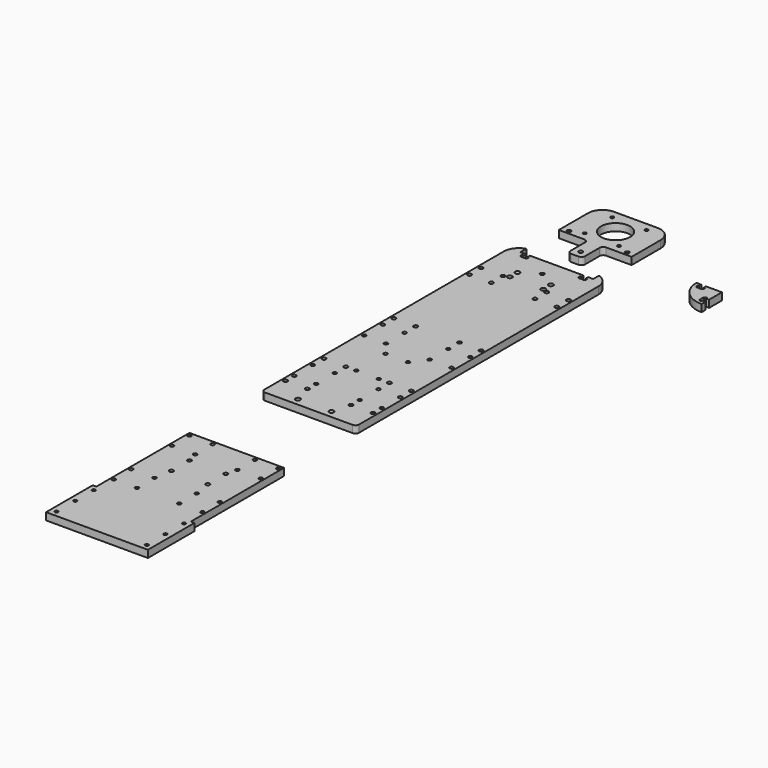
from build123d import *

# Parameters (mm, degrees)
F0_R     = 2.75
F0_R_2   = 2.5
F0_R_3   = 3.3
F1_DEPTH = 10
F0_W     = 130
F0_H     = 140
F0_H_2   = 20
F0_H_3   = 80
F0_R_4   = 2.25
F0_W_2   = 5
F2_DEPTH = 10
F0_R_5   = 20
F3_DEPTH = 10
F4_DEPTH = 10


# Not quite as in the source:
# - a feature names something its author has since deleted; it is built from what else it names


with BuildPart() as f1:
    # F0 (on Top) → F1 (new body)
    with BuildSketch(Plane.XY):
        with BuildLine():
            Line((65, 200), (-65, 200))
            Line((-65, 200), (-65, -121))
            ThreePointArc((-65, -121), (-63.5355339059, -124.5355339059), (-60, -126))
            Line((-60, -126), (60, -126))
            ThreePointArc((60, -126), (63.5355339059, -124.5355339059), (65, -121))
            Line((65, -121), (65, 200))
        make_face()
        with Locations((-60, -91)):
            Circle(F0_R, mode=Mode.SUBTRACT)
        with Locations((-60, -76)):
            Circle(F0_R_2, mode=Mode.SUBTRACT)
        with Locations((-60, -44)):
            Circle(F0_R_2, mode=Mode.SUBTRACT)
        with Locations((-30, -91)):
            Circle(F0_R, mode=Mode.SUBTRACT)
        with Locations((-23, -116)):
            Circle(F0_R_3, mode=Mode.SUBTRACT)
        with Locations((-30, -76)):
            Circle(F0_R_2, mode=Mode.SUBTRACT)
        with Locations((-30, -44)):
            Circle(F0_R_2, mode=Mode.SUBTRACT)
        with Locations((23, -116)):
            Circle(F0_R_3, mode=Mode.SUBTRACT)
        with Locations((30, -91)):
            Circle(F0_R, mode=Mode.SUBTRACT)
        with Locations((30, -76)):
            Circle(F0_R_2, mode=Mode.SUBTRACT)
        with Locations((30, -44)):
            Circle(F0_R_2, mode=Mode.SUBTRACT)
        with Locations((60, -91)):
            Circle(F0_R, mode=Mode.SUBTRACT)
        with Locations((60, -76)):
            Circle(F0_R_2, mode=Mode.SUBTRACT)
        with Locations((60, -44)):
            Circle(F0_R_2, mode=Mode.SUBTRACT)
        with Locations((-60, -25)):
            Circle(F0_R, mode=Mode.SUBTRACT)
        with Locations((-60, 44)):
            Circle(F0_R_2, mode=Mode.SUBTRACT)
        with Locations((-60, 76)):
            Circle(F0_R_2, mode=Mode.SUBTRACT)
        with Locations((-30, -25)):
            Circle(F0_R, mode=Mode.SUBTRACT)
        with Locations((-15.5, -25)):
            Circle(F0_R_2, mode=Mode.SUBTRACT)
        with Locations((-15.5, 25)):
            Circle(F0_R_2, mode=Mode.SUBTRACT)
        with Locations((-30, 44)):
            Circle(F0_R_2, mode=Mode.SUBTRACT)
        with Locations((-30, 76)):
            Circle(F0_R_2, mode=Mode.SUBTRACT)
        with Locations((-60, 95)):
            Circle(F0_R, mode=Mode.SUBTRACT)
        with Locations((-30, 95)):
            Circle(F0_R, mode=Mode.SUBTRACT)
        with Locations((15.5, -25)):
            Circle(F0_R_2, mode=Mode.SUBTRACT)
        with Locations((15.5, 25)):
            Circle(F0_R_2, mode=Mode.SUBTRACT)
        with Locations((30, -25)):
            Circle(F0_R, mode=Mode.SUBTRACT)
        with Locations((30, 44)):
            Circle(F0_R_2, mode=Mode.SUBTRACT)
        with Locations((30, 76)):
            Circle(F0_R_2, mode=Mode.SUBTRACT)
        with Locations((30, 95)):
            Circle(F0_R, mode=Mode.SUBTRACT)
        with Locations((60, -25)):
            Circle(F0_R, mode=Mode.SUBTRACT)
        with Locations((60, 44)):
            Circle(F0_R_2, mode=Mode.SUBTRACT)
        with Locations((60, 76)):
            Circle(F0_R_2, mode=Mode.SUBTRACT)
        with Locations((60, 95)):
            Circle(F0_R, mode=Mode.SUBTRACT)
        with BuildLine():
            Line((-65, 290), (-65, 200))
            Line((-65, 200), (65, 200))
            Line((65, 200), (65, 290))
            ThreePointArc((65, 290), (62.0710678119, 297.0710678119), (55, 300))
            Line((55, 300), (50, 300))
            Line((50, 300), (43, 300))
            Line((43, 300), (43, 296))
            Line((43, 296), (45, 296))
            Line((45, 296), (45, 293.6))
            Line((45, 293.6), (43.4, 292))
            Line((43.4, 292), (40, 292))
            Line((40, 292), (36.6, 292))
            Line((36.6, 292), (35, 293.6))
            Line((35, 293.6), (35, 296))
            Line((35, 296), (37, 296))
            Line((37, 296), (37, 300))
            Line((37, 300), (-37, 300))
            Line((-37, 300), (-37, 296))
            Line((-37, 296), (-35, 296))
            Line((-35, 296), (-35, 293.6))
            Line((-35, 293.6), (-36.6, 292))
            Line((-36.6, 292), (-37.5, 292))
            Line((-37.5, 292), (-40, 292))
            Line((-40, 292), (-42.5, 292))
            Line((-42.5, 292), (-43.4, 292))
            Line((-43.4, 292), (-45, 293.6))
            Line((-45, 293.6), (-45, 296))
            Line((-45, 296), (-43, 296))
            Line((-43, 296), (-43, 300))
            Line((-43, 300), (-50, 300))
            Line((-50, 300), (-55, 300))
            ThreePointArc((-55, 300), (-62.0710678119, 297.0710678119), (-65, 290))
        make_face()
        with Locations((-60, 225)):
            Circle(F0_R, mode=Mode.SUBTRACT)
        with Locations((-60, 245)):
            Circle(F0_R, mode=Mode.SUBTRACT)
        with Locations((-30, 225)):
            Circle(F0_R, mode=Mode.SUBTRACT)
        with Locations((-30, 245)):
            Circle(F0_R, mode=Mode.SUBTRACT)
        with Locations((-23, 248)):
            Circle(F0_R_3, mode=Mode.SUBTRACT)
        with Locations((-23, 261)):
            Circle(F0_R_3, mode=Mode.SUBTRACT)
        with Locations((0, 275)):
            Circle(F0_R, mode=Mode.SUBTRACT)
        with Locations((30, 225)):
            Circle(F0_R, mode=Mode.SUBTRACT)
        with Locations((30, 245)):
            Circle(F0_R, mode=Mode.SUBTRACT)
        with Locations((23, 248)):
            Circle(F0_R_3, mode=Mode.SUBTRACT)
        with Locations((23, 261)):
            Circle(F0_R_3, mode=Mode.SUBTRACT)
        with Locations((60, 225)):
            Circle(F0_R, mode=Mode.SUBTRACT)
        with Locations((60, 245)):
            Circle(F0_R, mode=Mode.SUBTRACT)
        with BuildLine():
            ThreePointArc((-50, 310), (-60.8333333333, 302.5), (-65, 290))
            ThreePointArc((-65, 290), (-62.0710678119, 297.0710678119), (-55, 300))
            Line((-55, 300), (-50, 300))
            Line((-50, 300), (-50, 310))
        make_face()
        with BuildLine():
            ThreePointArc((55, 300), (62.0710678119, 297.0710678119), (65, 290))
            ThreePointArc((65, 290), (60.8333333333, 302.5), (50, 310))
            Line((50, 310), (50, 300))
            Line((50, 300), (55, 300))
        make_face()
    extrude(amount=F1_DEPTH)


with BuildPart() as f2:
    # F0 (on Top) → F2 (new body)
    with BuildSketch(Plane.XY):
        with Locations((0, -320)):
            Rectangle(F0_W, F0_H)
        with Locations((-61, -385)):
            Circle(F0_R_2, mode=Mode.SUBTRACT)
        with Locations((-29, -385)):
            Circle(F0_R_2, mode=Mode.SUBTRACT)
        with Locations((-61, -355)):
            Circle(F0_R_2, mode=Mode.SUBTRACT)
        with Locations((-61, -285)):
            Circle(F0_R_2, mode=Mode.SUBTRACT)
        with Locations((-29, -355)):
            Circle(F0_R_2, mode=Mode.SUBTRACT)
        with Locations((-25, -331)):
            Circle(F0_R, mode=Mode.SUBTRACT)
        with Locations((-25, -300)):
            Circle(F0_R, mode=Mode.SUBTRACT)
        with Locations((-29, -285)):
            Circle(F0_R_2, mode=Mode.SUBTRACT)
        with Locations((29, -385)):
            Circle(F0_R_2, mode=Mode.SUBTRACT)
        with Locations((29, -355)):
            Circle(F0_R_2, mode=Mode.SUBTRACT)
        with Locations((25, -331)):
            Circle(F0_R, mode=Mode.SUBTRACT)
        with Locations((25, -300)):
            Circle(F0_R, mode=Mode.SUBTRACT)
        with Locations((29, -285)):
            Circle(F0_R_2, mode=Mode.SUBTRACT)
        with Locations((-61, -255)):
            Circle(F0_R_2, mode=Mode.SUBTRACT)
        with Locations((-29, -255)):
            Circle(F0_R_2, mode=Mode.SUBTRACT)
        with Locations((29, -255)):
            Circle(F0_R_2, mode=Mode.SUBTRACT)
        with Locations((61, -385)):
            Circle(F0_R_2, mode=Mode.SUBTRACT)
        with Locations((61, -355)):
            Circle(F0_R_2, mode=Mode.SUBTRACT)
        with Locations((61, -285)):
            Circle(F0_R_2, mode=Mode.SUBTRACT)
        with Locations((61, -255)):
            Circle(F0_R_2, mode=Mode.SUBTRACT)
        with Locations((0, -400)):
            Rectangle(F0_W, F0_H_2)
        with Locations((0, -450)):
            Rectangle(F0_W, F0_H_3)
        with Locations((-62, -482)):
            Circle(F0_R_4, mode=Mode.SUBTRACT)
        with Locations((-62, -450)):
            Circle(F0_R_4, mode=Mode.SUBTRACT)
        with Locations((-62, -418)):
            Circle(F0_R_4, mode=Mode.SUBTRACT)
        with Locations((62, -482)):
            Circle(F0_R_4, mode=Mode.SUBTRACT)
        with Locations((62, -450)):
            Circle(F0_R_4, mode=Mode.SUBTRACT)
        with Locations((62, -418)):
            Circle(F0_R_4, mode=Mode.SUBTRACT)
        with Locations((-67.5, -450)):
            Rectangle(F0_W_2, F0_H_3)
        with Locations((67.5, -450)):
            Rectangle(F0_W_2, F0_H_3)
    extrude(amount=F2_DEPTH)


with BuildPart() as f3:
    # F0 (on Top) → F3 (new body)
    with BuildSketch(Plane.XY):
        with BuildLine():
            Line((15, 366), (50, 366))
            Line((50, 366), (50, 416))
            ThreePointArc((50, 416), (44.1421356237, 430.1421356237), (30, 436))
            Line((30, 436), (-30, 436))
            ThreePointArc((-30, 436), (-44.1421356237, 430.1421356237), (-50, 416))
            Line((-50, 416), (-50, 366))
            Line((-50, 366), (-15, 366))
            ThreePointArc((-15, 366), (-11.4644660941, 364.5355339059), (-10, 361))
            Line((-10, 361), (-10, 336))
            ThreePointArc((-10, 336), (-8.5355339059, 332.4644660941), (-5, 331))
            Line((-5, 331), (5, 331))
            ThreePointArc((5, 331), (8.5355339059, 332.4644660941), (10, 336))
            Line((10, 336), (10, 361))
            ThreePointArc((10, 361), (11.4644660941, 364.5355339059), (15, 366))
        make_face()
        with Locations((-40, 371)):
            Circle(F0_R, mode=Mode.SUBTRACT)
        with Locations((-23.65, 377.35)):
            Circle(F0_R_4, mode=Mode.SUBTRACT)
        with Locations((-23.65, 424.65)):
            Circle(F0_R_4, mode=Mode.SUBTRACT)
        with Locations((0, 341)):
            Circle(F0_R, mode=Mode.SUBTRACT)
        with Locations((0, 401)):
            Circle(F0_R_5, mode=Mode.SUBTRACT)
        with Locations((23.65, 377.35)):
            Circle(F0_R_4, mode=Mode.SUBTRACT)
        with Locations((40, 371)):
            Circle(F0_R, mode=Mode.SUBTRACT)
        with Locations((23.65, 424.65)):
            Circle(F0_R_4, mode=Mode.SUBTRACT)
    extrude(amount=F3_DEPTH)


with BuildPart() as f4:
    # F0 (on Top) → F4 (new body)
    with BuildSketch(Plane.XY):
        with BuildLine():
            Line((154.638248086, 354.2600654125), (152.138248086, 354.2600654125))
            Line((152.138248086, 354.2600654125), (149.638248086, 354.2600654125))
            Line((149.638248086, 354.2600654125), (148.738248086, 354.2600654125))
            Line((148.738248086, 354.2600654125), (147.138248086, 355.8600654125))
            Line((147.138248086, 355.8600654125), (147.138248086, 358.2600654125))
            Line((147.138248086, 358.2600654125), (149.138248086, 358.2600654125))
            Line((149.138248086, 358.2600654125), (149.138248086, 362.2600654125))
            Line((149.138248086, 362.2600654125), (142.138248086, 362.2600654125))
            ThreePointArc((142.138248086, 362.2600654125), (152.3895107444, 337.511328071), (177.138248086, 327.2600654125))
            Line((177.138248086, 327.2600654125), (177.138248086, 334.2600654125))
            Line((177.138248086, 334.2600654125), (173.138248086, 334.2600654125))
            Line((173.138248086, 334.2600654125), (173.138248086, 332.2600654125))
            Line((173.138248086, 332.2600654125), (170.738248086, 332.2600654125))
            Line((170.738248086, 332.2600654125), (169.138248086, 333.8600654125))
            Line((169.138248086, 333.8600654125), (169.138248086, 334.7600654125))
            Line((169.138248086, 334.7600654125), (169.138248086, 337.2600654125))
            Line((169.138248086, 337.2600654125), (169.138248086, 339.7600654125))
            Line((169.138248086, 339.7600654125), (169.138248086, 340.6600654125))
            Line((169.138248086, 340.6600654125), (170.738248086, 342.2600654125))
            Line((170.738248086, 342.2600654125), (173.138248086, 342.2600654125))
            Line((173.138248086, 342.2600654125), (173.138248086, 340.2600654125))
            Line((173.138248086, 340.2600654125), (177.138248086, 340.2600654125))
            Line((177.138248086, 340.2600654125), (177.138248086, 362.2600654125))
            Line((177.138248086, 362.2600654125), (155.138248086, 362.2600654125))
            Line((155.138248086, 362.2600654125), (155.138248086, 358.2600654125))
            Line((155.138248086, 358.2600654125), (157.138248086, 358.2600654125))
            Line((157.138248086, 358.2600654125), (157.138248086, 355.8600654125))
            Line((157.138248086, 355.8600654125), (155.538248086, 354.2600654125))
            Line((155.538248086, 354.2600654125), (154.638248086, 354.2600654125))
        make_face()
    extrude(amount=F4_DEPTH)


solid = Compound([f1.part, f2.part, f3.part, f4.part])
